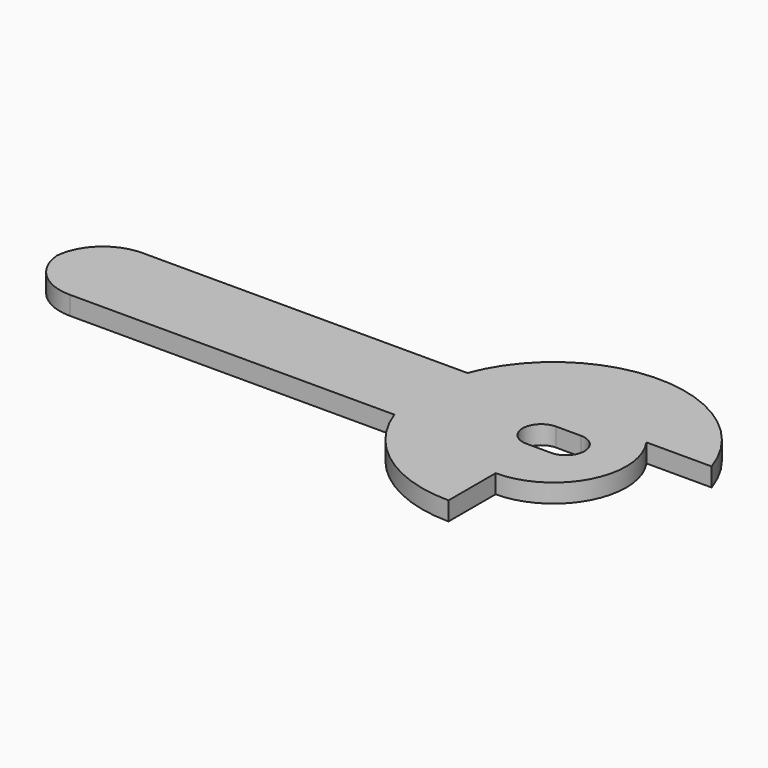
from build123d import *

# Parameters (mm, degrees)
F1_DEPTH    = 1.5
F3_DEPTH    = 3
F4_T1_DEPTH = 42.8345237792


# Not quite as in the source:
# - a fillet or chamfer that OpenCascade refuses, or shapes differently, is made with other operations: its cross-section is extruded or revolved along the edge and cut away or added


with BuildPart() as f1:
    # F0 (on Top) → F1 (new body, symmetric)
    with BuildSketch(Plane.XY):
        with BuildLine():
            Line((9.5752676601, 6.7411407109), (20.1104327648, 6.7411407109))
            ThreePointArc((20.1104327648, 6.7411407109), (-17.2170469432, 12.3873233035), (0, -21.2101976434))
            Line((0, -21.2101976434), (0, -11.7101976434))
            ThreePointArc((0, -11.7101976434), (10.3939602393, -5.3939150337), (9.5752676601, 6.7411407109))
        make_face()
        with BuildLine():
            Line((2, -3), (-2, -3))
            ThreePointArc((-2, -3), (-5, 0), (-2, 3))
            Line((-2, 3), (2, 3))
            ThreePointArc((2, 3), (5, 0), (2, -3))
        make_face(mode=Mode.SUBTRACT)
    extrude(amount=F1_DEPTH, both=True)

    # F2 (on face) → F3 (join)
    with BuildSketch(Plane.XY.offset(1.5)):
        with BuildLine():
            ThreePointArc((-19.9517186141, -7.19731953), (-21.2098366027, 0.1237552257), (-19.8663731217, 7.4296502651))
            Line((-19.8663731217, 7.4296502651), (-80.3057924461, 7.4296502651))
            Line((-80.3057924461, 7.4296502651), (-80.3057924461, -7.19731953))
            Line((-80.3057924461, -7.19731953), (-19.9517186141, -7.19731953))
        make_face()
    extrude(amount=-F3_DEPTH)

    # F4: fillet of radius 7.9669047558 on 2 edges, made by hand

    # F4_s2 → F4_t1 (cut)
    with BuildSketch(Plane.XY.offset(-21.4172618896)):
        with BuildLine():
            ThreePointArc((-72.3388876903, -7.19731953), (-77.9723400682, -4.863867152), (-80.3057924461, 0.7695852259))
            Line((-80.3057924461, 0.7695852259), (-80.3057924461, -7.19731953))
            Line((-80.3057924461, -7.19731953), (-72.3388876903, -7.19731953))
        make_face()
        with BuildLine():
            ThreePointArc((-72.3388876903, 7.4296502651), (-77.9723400682, 5.0961978872), (-80.3057924461, -0.5372544907))
            Line((-80.3057924461, -0.5372544907), (-80.3057924461, 7.4296502651))
            Line((-80.3057924461, 7.4296502651), (-72.3388876903, 7.4296502651))
        make_face()
    extrude(amount=F4_T1_DEPTH, mode=Mode.SUBTRACT)


solid = f1.part
